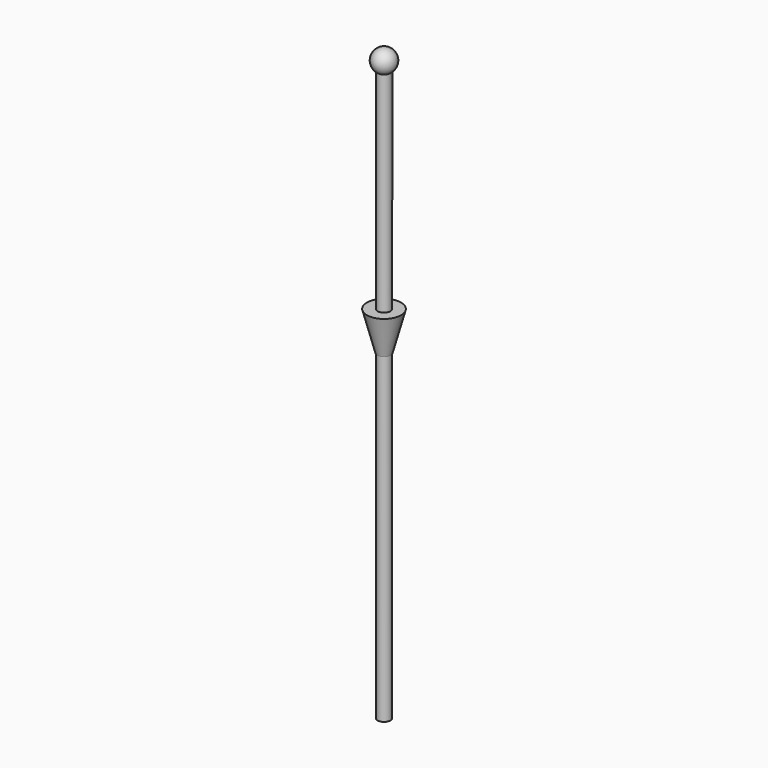
from build123d import *

# Parameters (mm, degrees)
F0_R                   = 1
F1_DEPTH               = 90
F5_R                   = 1.05
F5_R_2                 = 1
F6_DEPTH               = 6
DRAFT_F6_DRAFTED_ANGLE = -15


# Not quite as in the source:
# - an extrude with a draft is written as a straight extrude whose walls are then drafted


with BuildPart() as f1:
    # F0 (on Top) → F1 (new body)
    with BuildSketch(Plane.XY):
        with Locations((-2.7182325721, 0.6486773491)):
            Circle(F0_R)
    extrude(amount=F1_DEPTH)

    # F2 (on face) → F3 (revolve)
    with BuildSketch(Plane.XY.offset(90)):
        with BuildLine():
            ThreePointArc((-2.7182325721, -1.090586384), (-0.978968839, 0.6486773491), (-2.7182325721, 2.3879410821))
            Line((-2.7182325721, 2.3879410821), (-2.7182325721, 1.6486773491))
            ThreePointArc((-2.7182325721, 1.6486773491), (-2.0111257909, 1.3557841303), (-1.7182325721, 0.6486773491))
            ThreePointArc((-1.7182325721, 0.6486773491), (-2.0111257909, -0.0584294321), (-2.7182325721, -0.3513226509))
            Line((-2.7182325721, -0.3513226509), (-2.7182325721, -1.090586384))
        make_face()
        with BuildLine():
            ThreePointArc((-1.7182325721, 0.6486773491), (-2.0111257909, 1.3557841303), (-2.7182325721, 1.6486773491))
            Line((-2.7182325721, 1.6486773491), (-2.7182325721, -0.3513226509))
            ThreePointArc((-2.7182325721, -0.3513226509), (-2.0111257909, -0.0584294321), (-1.7182325721, 0.6486773491))
        make_face()
    revolve(axis=Axis((-2.7182325721, 0.6486773491, 90), (0, -1, 0)))


with BuildPart() as f6_drafted:
    # F5 (on offset) → F6 (new body)
    with BuildSketch(Plane.XY.offset(50)):
        with Locations((-2.7182325721, 0.6486773491)):
            Circle(F5_R)
        with Locations((-2.7182325721, 0.6486773491)):
            Circle(F5_R_2, mode=Mode.SUBTRACT)
    extrude(amount=F6_DEPTH)

    # draft_F6_drafted
    draft_f6_drafted_walls = [f6_drafted.faces().sort_by_distance(p)[0] for p in [
        (-3.7682325721, 0.6486773491, 54),
        (-3.7182325721, 0.6486773491, 54),
    ]]
    draft(draft_f6_drafted_walls, neutral_plane=Plane.XY.offset(50), angle=DRAFT_F6_DRAFTED_ANGLE)


with BuildPart() as f1_1:
    add(f1.part)

    # join_F6_drafted: union F6_drafted
    add(f6_drafted.part)


solid = f1_1.part
